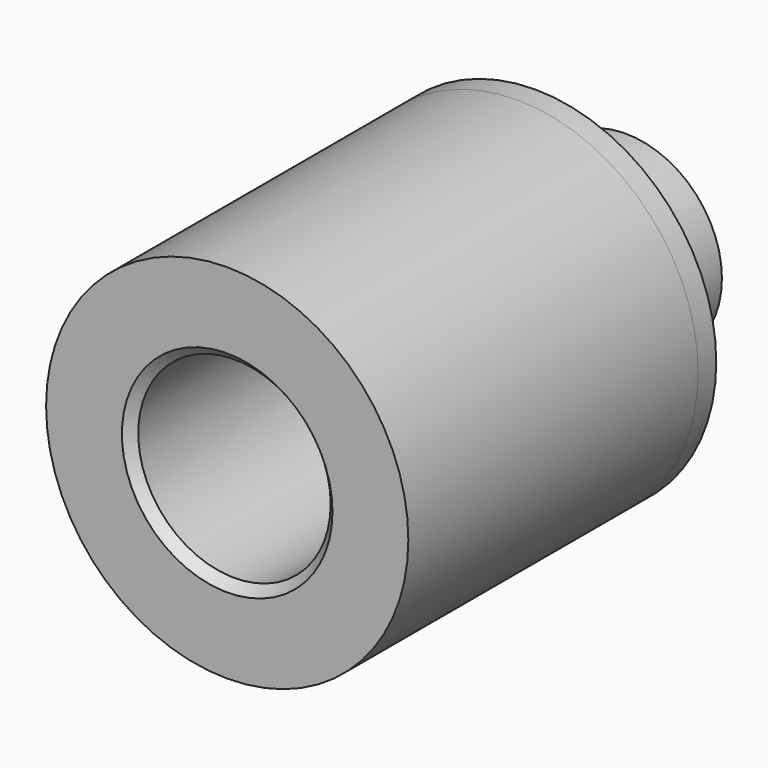
from build123d import *

# Parameters (mm, degrees)
F0_R     = 26.9875
F1_DEPTH = 38.1
F0_R_2   = 50.8
F2_DEPTH = 6.35
F3_DEPTH = 101.6
F4_R     = 24.5602140896
F5_DEPTH = 127
F6_SIZE2 = 2.54
F6_SIZE  = 2.54
F7_T     = -2.54


# Not quite as in the source:
# - a feature names something its author has since deleted; it is built from what else it names


with BuildPart() as f1:
    # F0 (on Front) → F1 (new body)
    with BuildSketch(Plane.XZ):
        Circle(F0_R)
    extrude(amount=-F1_DEPTH)

    # F0 (on Front) → F2 (join)
    with BuildSketch(Plane.XZ):
        Circle(F0_R_2)
        Circle(F0_R, mode=Mode.SUBTRACT)
    extrude(amount=-F2_DEPTH)

    # F0 (on Front) → F3 (join)
    with BuildSketch(Plane.XZ):
        Circle(F0_R_2)
        Circle(F0_R, mode=Mode.SUBTRACT)
    extrude(amount=F3_DEPTH)

    # F4 (on face) → F5 (cut)
    with BuildSketch(Plane(origin=(0, 38.1, 0), x_dir=(-1, 0, 0), z_dir=(0, 1, 0))):
        Circle(F4_R)
    extrude(amount=-F5_DEPTH, mode=Mode.SUBTRACT)

    # F6
    f6_edges = [f1.edges().sort_by_distance(p)[0] for p in [
        (-26.9875, -101.6, 0),
    ]]
    chamfer(f6_edges, length=F6_SIZE, length2=F6_SIZE2)

    # F7 (hollow: no face is removed)
    offset(amount=F7_T, kind=Kind.INTERSECTION, mode=Mode.SUBTRACT)


solid = f1.part
